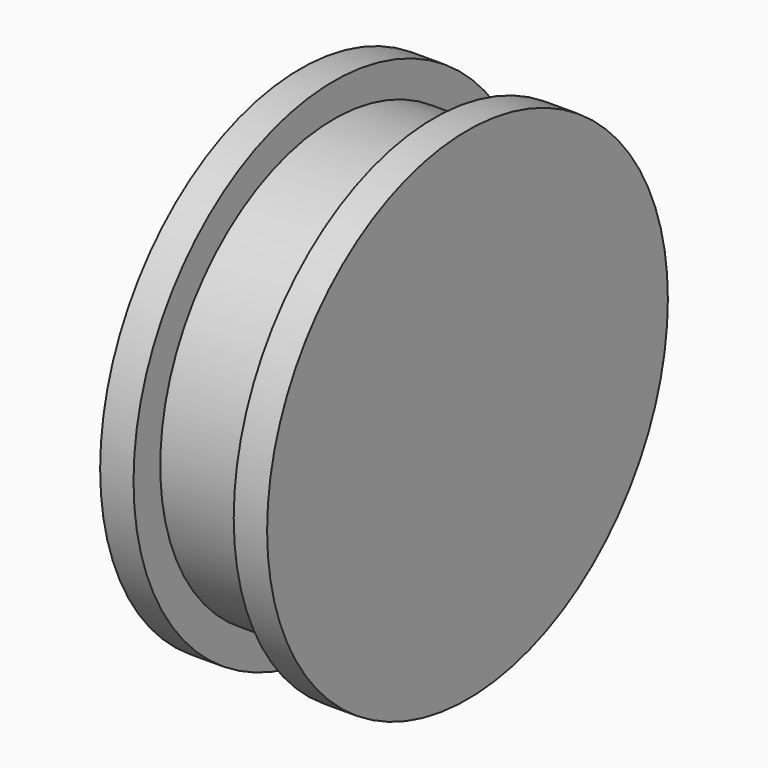
from build123d import *

# Parameters (mm, degrees)
F0_R     = 15
F1_DEPTH = 5
F2_R     = 15
F2_R_2   = 13
F3_DEPTH = 3


# Not quite as in the source:
# - a feature names something its author has since deleted; it is built from what else it names


with BuildPart() as f1:
    # F0 (on Right) → F1 (new body, symmetric)
    with BuildSketch(Plane.YZ):
        Circle(F0_R)
    extrude(amount=F1_DEPTH, both=True)

    # F2 (on Right) → F3 (cut, symmetric)
    with BuildSketch(Plane.YZ):
        Circle(F2_R)
        Circle(F2_R_2, mode=Mode.SUBTRACT)
    extrude(amount=F3_DEPTH, both=True, mode=Mode.SUBTRACT)


solid = f1.part
